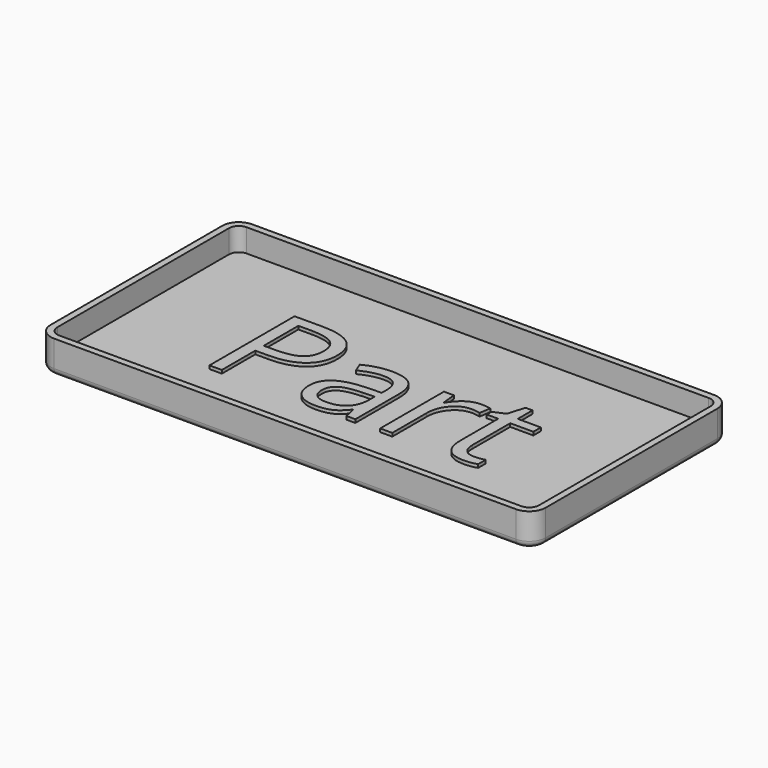
from build123d import *

# Parameters (mm, degrees)
F1_DEPTH     = 3
F2_DEPTH     = 10
F0_TEXT_SIZE = 45.1388888889
F3_DEPTH     = 4
F4_R         = 2


# Not quite as in the source:
# - Text() gives the source's letters only with a copy of the font that has no kerning and outlines rounded to 1/6400 em; it was checked with that copy


with BuildPart() as f1:
    # F0 (on Top) → F1 (new body)
    with BuildSketch(Plane.XY):
        with BuildLine():
            ThreePointArc((-44.6118305922, 5), (-43.7331509357, 2.8786796564), (-41.6118305922, 2))
            Line((-41.6118305922, 2), (98.3881694078, 2))
            ThreePointArc((98.3881694078, 2), (100.5094897514, 2.8786796564), (101.3881694078, 5))
            Line((101.3881694078, 5), (101.3881694078, 70))
            ThreePointArc((101.3881694078, 70), (100.5094897514, 72.1213203436), (98.3881694078, 73))
            Line((98.3881694078, 73), (-41.6118305922, 73))
            ThreePointArc((-41.6118305922, 73), (-43.7331509357, 72.1213203436), (-44.6118305922, 70))
            Line((-44.6118305922, 70), (-44.6118305922, 5))
        make_face()
        with BuildLine():
            add(Edge.make_bspline(
                [(-3.1349968248, 53.4749348958), (8.939655953, 53.4749348958), (8.939655953, 44.0874565972)],
                knots=[0, 0, 0, 1, 1, 1], degree=2))
            add(Edge.make_bspline(
                [(8.939655953, 44.0874565972), (8.939655953, 39.1927083333), (5.6000834703, 36.5584309896)],
                knots=[0, 0, 0, 1, 1, 1], degree=2))
            add(Edge.make_bspline(
                [(5.6000834703, 36.5584309896), (2.2605109877, 33.9241536458), (-3.9531391859, 33.9241536458)],
                knots=[0, 0, 0, 1, 1, 1], degree=2))
            Line((-3.9531391859, 33.9241536458), (-7.7476270331, 33.9241536458))
            Line((-7.7476270331, 33.9241536458), (-7.7476270331, 21.25))
            Line((-7.7476270331, 21.25), (-11.4927442206, 21.25))
            Line((-11.4927442206, 21.25), (-11.4927442206, 53.4749348958))
            Line((-11.4927442206, 53.4749348958), (-3.1349968248, 53.4749348958))
        make_face(mode=Mode.SUBTRACT)
        with BuildLine():
            Line((32.7010491822, 21.25), (29.9856628974, 21.25))
            Line((29.9856628974, 21.25), (29.2592089044, 24.6918402778))
            Line((29.2592089044, 24.6918402778), (29.0828851197, 24.6918402778))
            add(Edge.make_bspline(
                [(29.0828851197, 24.6918402778), (27.2773295641, 22.4207899306), (25.4823534356, 21.6132269965)],
                knots=[0, 0, 0, 1, 1, 1], degree=2))
            add(Edge.make_bspline(
                [(25.4823534356, 21.6132269965), (23.6873773072, 20.8056640625), (20.9931498766, 20.8056640625)],
                knots=[0, 0, 0, 1, 1, 1], degree=2))
            add(Edge.make_bspline(
                [(20.9931498766, 20.8056640625), (17.4031976197, 20.8056640625), (15.3648946683, 22.6605902778)],
                knots=[0, 0, 0, 1, 1, 1], degree=2))
            add(Edge.make_bspline(
                [(15.3648946683, 22.6605902778), (13.3265917169, 24.5155164931), (13.3265917169, 27.9291449653)],
                knots=[0, 0, 0, 1, 1, 1], degree=2))
            add(Edge.make_bspline(
                [(13.3265917169, 27.9291449653), (13.3265917169, 35.2430555556), (25.027438071, 35.595703125)],
                knots=[0, 0, 0, 1, 1, 1], degree=2))
            Line((25.027438071, 35.595703125), (29.125202828, 35.7297092014))
            Line((29.125202828, 35.7297092014), (29.125202828, 37.2319878472))
            add(Edge.make_bspline(
                [(29.125202828, 37.2319878472), (29.125202828, 40.0743272569), (27.9050422377, 41.4284939236)],
                knots=[0, 0, 0, 1, 1, 1], degree=2))
            add(Edge.make_bspline(
                [(27.9050422377, 41.4284939236), (26.6848816474, 42.7826605903), (23.9906542169, 42.7826605903)],
                knots=[0, 0, 0, 1, 1, 1], degree=2))
            add(Edge.make_bspline(
                [(23.9906542169, 42.7826605903), (20.9719910224, 42.7826605903), (17.1633972724, 40.9347873264)],
                knots=[0, 0, 0, 1, 1, 1], degree=2))
            Line((17.1633972724, 40.9347873264), (16.0349250502, 43.7348090278))
            add(Edge.make_bspline(
                [(16.0349250502, 43.7348090278), (17.8193217516, 44.7010633681), (19.9457865953, 45.2511935764)],
                knots=[0, 0, 0, 1, 1, 1], degree=2))
            add(Edge.make_bspline(
                [(19.9457865953, 45.2511935764), (22.0722514391, 45.8013237847), (24.2163486613, 45.8013237847)],
                knots=[0, 0, 0, 1, 1, 1], degree=2))
            add(Edge.make_bspline(
                [(24.2163486613, 45.8013237847), (28.5327549113, 45.8013237847), (30.6169020467, 43.8864474826)],
                knots=[0, 0, 0, 1, 1, 1], degree=2))
            add(Edge.make_bspline(
                [(30.6169020467, 43.8864474826), (32.7010491822, 41.9715711806), (32.7010491822, 37.7398003472)],
                knots=[0, 0, 0, 1, 1, 1], degree=2))
            Line((32.7010491822, 37.7398003472), (32.7010491822, 21.25))
        make_face(mode=Mode.SUBTRACT)
        with BuildLine():
            add(Edge.make_bspline(
                [(47.0890700155, 44.5705837674), (48.9863139391, 45.8506944444), (51.2573642863, 45.8506944444)],
                knots=[0, 0, 0, 1, 1, 1], degree=2))
            add(Edge.make_bspline(
                [(51.2573642863, 45.8506944444), (52.865437203, 45.8506944444), (54.1420214044, 45.5826822917)],
                knots=[0, 0, 0, 1, 1, 1], degree=2))
            Line((54.1420214044, 45.5826822917), (53.6342089044, 42.1902126736))
            add(Edge.make_bspline(
                [(53.6342089044, 42.1902126736), (52.1389832099, 42.5217013889), (50.9893521335, 42.5217013889)],
                knots=[0, 0, 0, 1, 1, 1], degree=2))
            add(Edge.make_bspline(
                [(50.9893521335, 42.5217013889), (48.0553243558, 42.5217013889), (45.974703696, 40.1413302951)],
                knots=[0, 0, 0, 1, 1, 1], degree=2))
            add(Edge.make_bspline(
                [(45.974703696, 40.1413302951), (43.8940830363, 37.7609592014), (43.8940830363, 34.2133246528)],
                knots=[0, 0, 0, 1, 1, 1], degree=2))
            Line((43.8940830363, 34.2133246528), (43.8940830363, 21.25))
            Line((43.8940830363, 21.25), (40.2336012655, 21.25))
            Line((40.2336012655, 21.25), (40.2336012655, 45.4063585069))
            Line((40.2336012655, 45.4063585069), (43.2522644599, 45.4063585069))
            Line((43.2522644599, 45.4063585069), (43.6754415433, 40.9347873264))
            Line((43.6754415433, 40.9347873264), (43.851765328, 40.9347873264))
            add(Edge.make_bspline(
                [(43.851765328, 40.9347873264), (45.1918260919, 43.2904730903), (47.0890700155, 44.5705837674)],
                knots=[0, 0, 0, 1, 1, 1], degree=2))
        make_face(mode=Mode.SUBTRACT)
        with BuildLine():
            add(Edge.make_bspline(
                [(63.621188071, 24.9986436632), (64.6579719252, 23.8313802083), (66.4635274808, 23.8313802083)],
                knots=[0, 0, 0, 1, 1, 1], degree=2))
            add(Edge.make_bspline(
                [(66.4635274808, 23.8313802083), (67.4368347724, 23.8313802083), (68.3396125502, 23.9724392361)],
                knots=[0, 0, 0, 1, 1, 1], degree=2))
            add(Edge.make_bspline(
                [(68.3396125502, 23.9724392361), (69.242390328, 24.1134982639), (69.7713616822, 24.2686631944)],
                knots=[0, 0, 0, 1, 1, 1], degree=2))
            Line((69.7713616822, 24.2686631944), (69.7713616822, 21.4686414931))
            add(Edge.make_bspline(
                [(69.7713616822, 21.4686414931), (69.1789137655, 21.1865234375), (68.0222297377, 20.99609375)],
                knots=[0, 0, 0, 1, 1, 1], degree=2))
            add(Edge.make_bspline(
                [(68.0222297377, 20.99609375), (66.8655457099, 20.8056640625), (65.9345561266, 20.8056640625)],
                knots=[0, 0, 0, 1, 1, 1], degree=2))
            add(Edge.make_bspline(
                [(65.9345561266, 20.8056640625), (58.9309753974, 20.8056640625), (58.9309753974, 28.1901041667)],
                knots=[0, 0, 0, 1, 1, 1], degree=2))
            Line((58.9309753974, 28.1901041667), (58.9309753974, 42.5640190972))
            Line((58.9309753974, 42.5640190972), (55.4679762655, 42.5640190972))
            Line((55.4679762655, 42.5640190972), (55.4679762655, 44.3272569444))
            Line((55.4679762655, 44.3272569444), (58.9309753974, 45.8506944444))
            Line((58.9309753974, 45.8506944444), (60.4685188002, 51.0064019097))
            Line((60.4685188002, 51.0064019097), (62.5844042169, 51.0064019097))
            Line((62.5844042169, 51.0064019097), (62.5844042169, 45.4063585069))
            Line((62.5844042169, 45.4063585069), (69.5950378974, 45.4063585069))
            Line((69.5950378974, 45.4063585069), (69.5950378974, 42.5640190972))
            Line((69.5950378974, 42.5640190972), (62.5844042169, 42.5640190972))
            Line((62.5844042169, 42.5640190972), (62.5844042169, 28.3452690972))
            add(Edge.make_bspline(
                [(62.5844042169, 28.3452690972), (62.5844042169, 26.1659071181), (63.621188071, 24.9986436632)],
                knots=[0, 0, 0, 1, 1, 1], degree=2))
        make_face(mode=Mode.SUBTRACT)
    extrude(amount=F1_DEPTH)

    # F0 (on Top) → F2 (join)
    with BuildSketch(Plane.XY):
        with BuildLine():
            Line((98.3881694078, 75), (-41.6118305922, 75))
            ThreePointArc((-41.6118305922, 75), (-45.1473644981, 73.5355339059), (-46.6118305922, 70))
            Line((-46.6118305922, 70), (-46.6118305922, 5))
            ThreePointArc((-46.6118305922, 5), (-45.1473644981, 1.4644660941), (-41.6118305922, 0))
            Line((-41.6118305922, 0), (98.3881694078, 0))
            ThreePointArc((98.3881694078, 0), (101.9237033138, 1.4644660941), (103.3881694078, 5))
            Line((103.3881694078, 5), (103.3881694078, 70))
            ThreePointArc((103.3881694078, 70), (101.9237033138, 73.5355339059), (98.3881694078, 75))
        make_face()
        with BuildLine():
            Line((98.3881694078, 2), (-41.6118305922, 2))
            ThreePointArc((-41.6118305922, 2), (-43.7331509357, 2.8786796564), (-44.6118305922, 5))
            Line((-44.6118305922, 5), (-44.6118305922, 70))
            ThreePointArc((-44.6118305922, 70), (-43.7331509357, 72.1213203436), (-41.6118305922, 73))
            Line((-41.6118305922, 73), (98.3881694078, 73))
            ThreePointArc((98.3881694078, 73), (100.5094897514, 72.1213203436), (101.3881694078, 70))
            Line((101.3881694078, 70), (101.3881694078, 5))
            ThreePointArc((101.3881694078, 5), (100.5094897514, 2.8786796564), (98.3881694078, 2))
        make_face(mode=Mode.SUBTRACT)
    extrude(amount=F2_DEPTH)



with BuildPart() as f1b:
    # F0 (on Top) → F1, piece 2 (new body)
    with BuildSketch(Plane.XY):
        with BuildLine():
            add(Edge.make_bspline(
                [(18.3623990085, 24.8646375868), (19.5614007447, 23.8313802083), (21.7196038697, 23.8313802083)],
                knots=[0, 0, 0, 1, 1, 1], degree=2))
            add(Edge.make_bspline(
                [(21.7196038697, 23.8313802083), (25.1402852933, 23.8313802083), (27.0904263523, 25.7039388021)],
                knots=[0, 0, 0, 1, 1, 1], degree=2))
            add(Edge.make_bspline(
                [(27.0904263523, 25.7039388021), (29.0405674113, 27.5764973958), (29.0405674113, 30.9478081597)],
                knots=[0, 0, 0, 1, 1, 1], degree=2))
            Line((29.0405674113, 30.9478081597), (29.0405674113, 33.1271701389))
            Line((29.0405674113, 33.1271701389), (25.3800856405, 32.9790581597))
            add(Edge.make_bspline(
                [(25.3800856405, 32.9790581597), (21.0143087308, 32.8238932292), (19.0888530016, 31.6213650174)],
                knots=[0, 0, 0, 1, 1, 1], degree=2))
            add(Edge.make_bspline(
                [(19.0888530016, 31.6213650174), (17.1633972724, 30.4188368056), (17.1633972724, 27.8868272569)],
                knots=[0, 0, 0, 1, 1, 1], degree=2))
            add(Edge.make_bspline(
                [(17.1633972724, 27.8868272569), (17.1633972724, 25.8978949653), (18.3623990085, 24.8646375868)],
                knots=[0, 0, 0, 1, 1, 1], degree=2))
        make_face()
    extrude(amount=F1_DEPTH)


with BuildPart() as f1c:
    # F0 (on Top) → F1, piece 3 (new body)
    with BuildSketch(Plane.XY):
        with BuildLine():
            Line((-7.7476270331, 50.2305772569), (-7.7476270331, 37.1402994792))
            Line((-7.7476270331, 37.1402994792), (-4.3692633178, 37.1402994792))
            add(Edge.make_bspline(
                [(-4.3692633178, 37.1402994792), (0.6101203627, 37.1402994792), (2.8353265259, 38.7483723958)],
                knots=[0, 0, 0, 1, 1, 1], degree=2))
            add(Edge.make_bspline(
                [(2.8353265259, 38.7483723958), (5.0605326891, 40.3564453125), (5.0605326891, 43.9111328125)],
                knots=[0, 0, 0, 1, 1, 1], degree=2))
            add(Edge.make_bspline(
                [(5.0605326891, 43.9111328125), (5.0605326891, 47.1061197917), (2.9658061266, 48.6683485243)],
                knots=[0, 0, 0, 1, 1, 1], degree=2))
            add(Edge.make_bspline(
                [(2.9658061266, 48.6683485243), (0.8710795641, 50.2305772569), (-3.5581739081, 50.2305772569)],
                knots=[0, 0, 0, 1, 1, 1], degree=2))
            Line((-3.5581739081, 50.2305772569), (-7.7476270331, 50.2305772569))
        make_face()
    extrude(amount=F1_DEPTH)


with BuildPart() as f1_1:
    add(f1.part)

    add(f1b.part)  # F3 merges F1b

    add(f1c.part)  # F3 merges F1c
    # F0 (on Top) → F3 (join)
    with BuildSketch(Plane.XY):
        with Locations((-15.9219976928, 21.25)):
            Text('Part', F0_TEXT_SIZE, font='Open Sans', text_align=(TextAlign.LEFT, TextAlign.BOTTOM))
    extrude(amount=F3_DEPTH)

    # F4
    f4_edges = [f1_1.edges().sort_by_distance(p)[0] for p in [
        (103.388169, 37.5, 0),
    ]]
    fillet(f4_edges, radius=F4_R)


solid = f1_1.part
